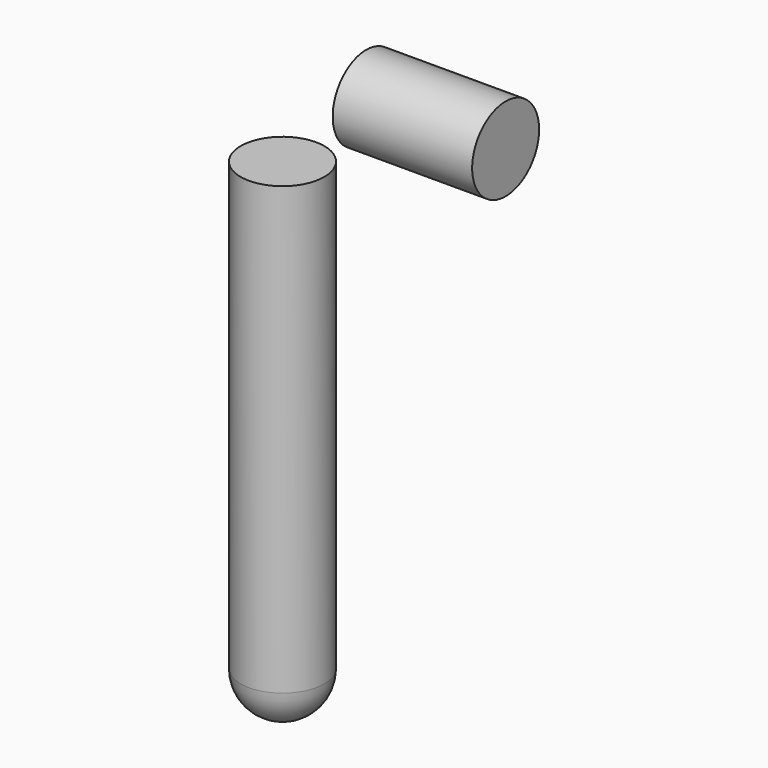
from build123d import *

# Parameters (mm, degrees)
F4_R     = 0.075
F5_DEPTH = 0.25


# Not quite as in the source:
# - the program builds the solid bodies; features that only make, move or delete a surface that nothing else refers to are left out


with BuildPart() as f1:
    # F0 (on Front) → F1 (revolve)
    with BuildSketch(Plane.XZ):
        with BuildLine():
            Line((0.075, 0), (0, 0))
            Line((0, 0), (0, -0.875))
            ThreePointArc((0, -0.875), (0.0530330086, -0.8530330086), (0.075, -0.8))
            Line((0.075, -0.8), (0.075, 0))
        make_face()
    revolve(axis=Axis((0, 0, -0.4375), (0, 0, -1)))


with BuildPart() as f5:
    # F4 (on offset) → F5 (new body)
    with BuildSketch(Plane.YZ.offset(0.15)):
        with Locations((0, 0.15)):
            Circle(F4_R)
    extrude(amount=F5_DEPTH)


solid = Compound([f1.part, f5.part])
